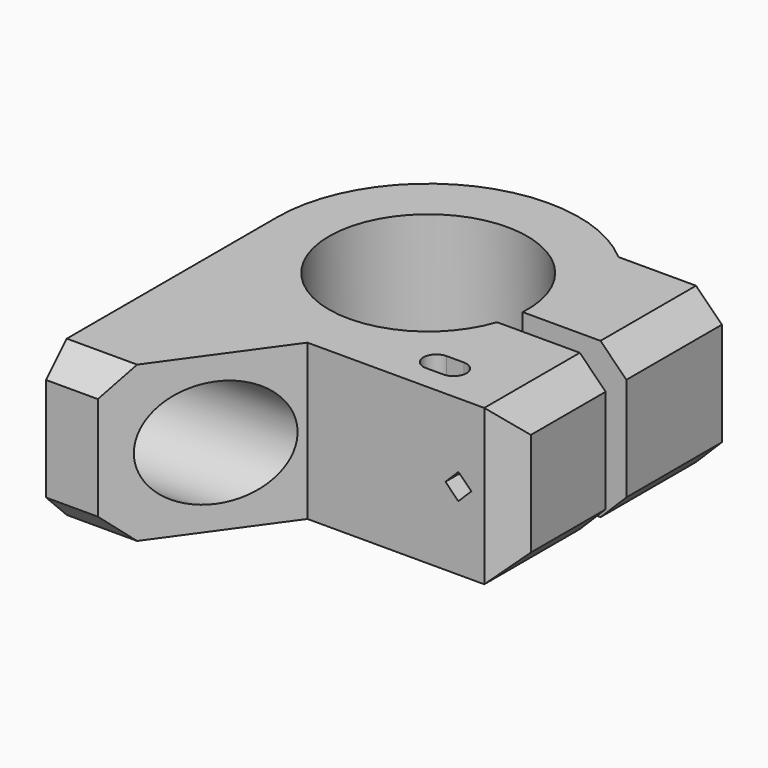
from build123d import *

# Parameters (mm, degrees)
F0_R     = 11.5
F1_DEPTH = 18
F2_R     = 6.25
F3_DEPTH = 41.001
F4_R     = 4.5
F5_DEPTH = 3
F6_SIZE  = 2.99999
F7_DEPTH = 46.6919059583
F9_DEPTH = 18.001
F10_SIZE = 3
F11_SIZE = 3


# Not quite as in the source:
# - a fillet or chamfer is up to 0.001 mm smaller than in the source, because OpenCascade refuses the exact size


with BuildPart() as f1:
    # F0 (on Top) → F1 (new body)
    with BuildSketch(Plane.XY):
        with BuildLine():
            Line((-17.5, 0), (-17.5, -33.5))
            Line((-17.5, -33.5), (-11.5, -33.5))
            Line((-11.5, -33.5), (0, -17.5))
            Line((0, -17.5), (23.5, -17.5))
            Line((23.5, -17.5), (23.5, -13.1909059583))
            Line((23.5, -13.1909059583), (23.5, 13.1909059583))
            Line((23.5, 13.1909059583), (11.5, 13.1909059583))
            ThreePointArc((11.5, 13.1909059583), (-7.2456883731, 15.9295323221), (-17.5, 0))
        make_face()
        with BuildLine():
            Line((13.5, -14.6909059583), (11.5, -14.6909059583))
            ThreePointArc((11.5, -14.6909059583), (10, -13.1909059583), (11.5, -11.6909059583))
            Line((11.5, -11.6909059583), (13.5, -11.6909059583))
            ThreePointArc((13.5, -11.6909059583), (15, -13.1909059583), (13.5, -14.6909059583))
        make_face(mode=Mode.SUBTRACT)
        Circle(F0_R, mode=Mode.SUBTRACT)
    extrude(amount=F1_DEPTH)

    # F2 (on face) → F3 (cut, through all)
    with BuildSketch(Plane(origin=(-17.5, 0, 0), x_dir=(0, -1, 0), z_dir=(-1, 0, 0))):
        with Locations((24.5, 9)):
            Circle(F2_R)
    extrude(amount=-F3_DEPTH, mode=Mode.SUBTRACT)

    # F4 (on face) → F5 (cut)
    with BuildSketch(Plane(origin=(0, 13.1909059583, 0), x_dir=(-1, 0, 0), z_dir=(0, 1, 0))):
        with Locations((-17.5, 9)):
            Circle(F4_R)
        Polygon((-19, 9), (-17.5, 10.5), (-16, 9), (-17.5, 7.5), align=None, mode=Mode.SUBTRACT)
    extrude(amount=-F5_DEPTH, mode=Mode.SUBTRACT)

    # F6 (size 3 in the source; OpenCascade refuses exactly that, so slightly less here)
    f6_edges = [f1.edges().sort_by_distance(p)[0] for p in [
        (22, 10.190906, 9),
    ]]
    chamfer(f6_edges, length=F6_SIZE)

    # F7 (cut, through all): a face of the model
    f7_faces = [f1.faces().sort_by_distance(p)[0] for p in [
        (17.5, 13.1909059583, 9),
    ]]
    extrude(f7_faces, amount=-F7_DEPTH, mode=Mode.SUBTRACT)

    # F8 (on face) → F9 (cut, through all)
    with BuildSketch(Plane(origin=(0, 0, 0), x_dir=(1, 0, 0), z_dir=(0, 0, -1))):
        with BuildLine():
            Line((23.5, 0.6545470209), (23.5, 3.6545470209))
            Line((23.5, 3.6545470209), (10.9038656481, 3.6545470209))
            ThreePointArc((10.9038656481, 3.6545470209), (11.2926769611, 2.1738093411), (11.4813574196, 0.6545470209))
            Line((11.4813574196, 0.6545470209), (23.5, 0.6545470209))
        make_face()
    extrude(amount=-F9_DEPTH, mode=Mode.SUBTRACT)

    # F10
    f10_edges = [f1.edges().sort_by_distance(p)[0] for p in [
        (23.5, 6.268179, 0),
        (23.5, 6.268179, 18),
        (23.5, -10.577274, 0),
        (23.5, -10.577274, 18),
        (23.5, -17.5, 9),
    ]]
    chamfer(f10_edges, length=F10_SIZE)

    # F11
    f11_edges = [f1.edges().sort_by_distance(p)[0] for p in [
        (-14.5, -33.5, 18),
        (-14.5, -33.5, 0),
    ]]
    chamfer(f11_edges, length=F11_SIZE)


solid = f1.part
